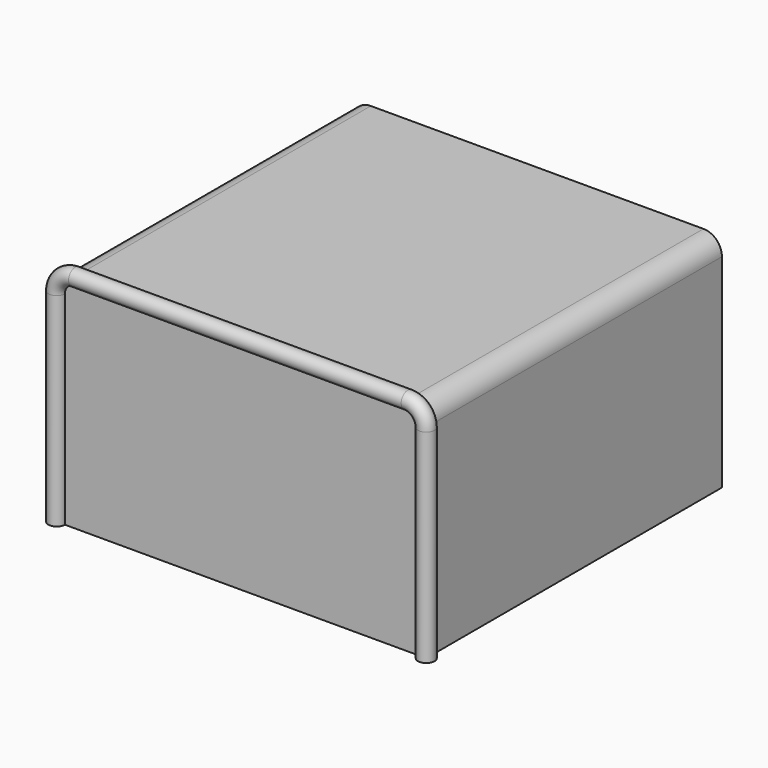
from build123d import *

# Parameters (mm, degrees)
F0_W     = 1000
F0_H     = 600
F1_DEPTH = 1000
F2_R     = 50
F3_R     = 50


with BuildPart() as f1:
    # F0 (on Front) → F1 (new body)
    with BuildSketch(Plane.XZ):
        with Locations((66.8085864745, -99.2259835054)):
            Rectangle(F0_W, F0_H)
    extrude(amount=F1_DEPTH)

    # F2
    f2_edges = [f1.edges().sort_by_distance(p)[0] for p in [
        (-433.191414, -500, 200.774016),
    ]]
    fillet(f2_edges, radius=F2_R)

    # F3
    f3_edges = [f1.edges().sort_by_distance(p)[0] for p in [
        (566.808586, -500, 200.774016),
    ]]
    fillet(f3_edges, radius=F3_R)

    # F5: sweep along a path in F5_path
    with BuildLine(Plane(origin=(-433.1914135255, -1000, -399.2259835054), x_dir=(0, 0, 1), z_dir=(0, -1, 0))) as f5_path:
        Line((0, 0), (550, 0))
        ThreePointArc((550, 0), (585.3553390593, -14.6446609407), (600, -50))
        Line((600, -50), (600, -950))
        ThreePointArc((600, -950), (585.3553390593, -985.3553390593), (550, -1000))
        Line((550, -1000), (0, -1000))
    # F4 (on face) → F5 (sweep)
    with BuildSketch(Plane(origin=(0, 0, -399.2259835054), x_dir=(1, 0, 0), z_dir=(0, 0, -1))):
        with BuildLine():
            ThreePointArc((-433.1914135255, 977.6715629095), (-417.4028242455, 984.21141072), (-410.862976435, 1000))
            Line((-410.862976435, 1000), (-433.1914135255, 1000))
            Line((-433.1914135255, 1000), (-433.1914135255, 977.6715629095))
        make_face()
        with BuildLine():
            Line((-433.1914135255, 1000), (-410.862976435, 1000))
            ThreePointArc((-410.862976435, 1000), (-448.9800028055, 1015.78858928), (-433.1914135255, 977.6715629095))
            Line((-433.1914135255, 977.6715629095), (-433.1914135255, 1000))
        make_face()
    sweep(path=f5_path.line)


solid = f1.part
